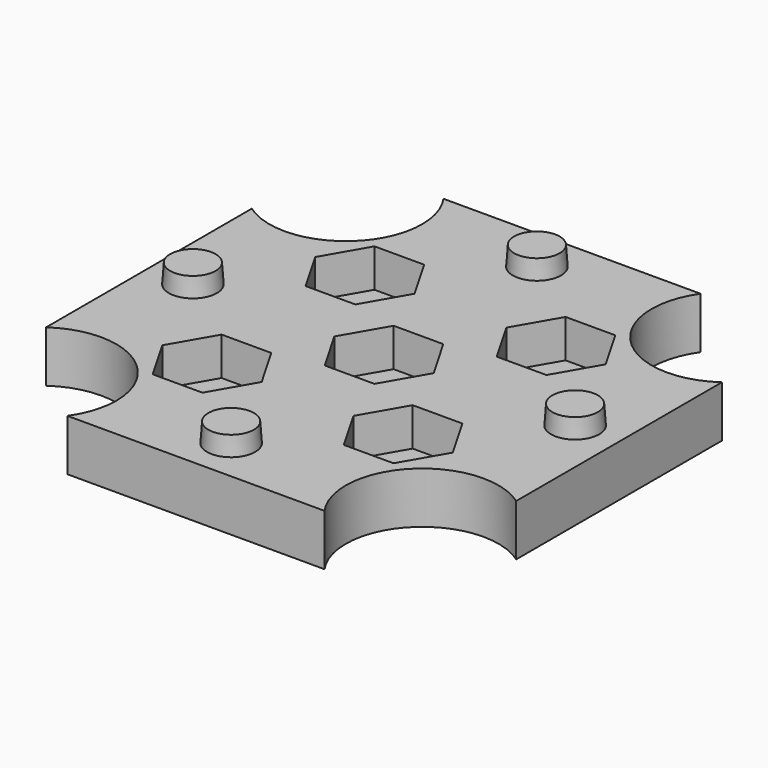
from build123d import *

# Parameters (mm, degrees)
F0_R       = 3.2004
F0_R_2     = 6.858
F1_DEPTH   = 6.8326
F2_DEPTH   = 9.3726
F3_R       = 3.2004
F4_DEPTH   = 5.08
F5_SIZE2   = 2.53999
F5_SIZE    = 0.17779
F5_2_SIZE2 = 2.53999
F5_2_SIZE  = 0.17779
F5_3_SIZE2 = 2.53999
F5_3_SIZE  = 0.17779
F5_4_SIZE2 = 2.53999
F5_4_SIZE  = 0.17779


# Not quite as in the source:
# - a fillet or chamfer is up to 0.001 mm smaller than in the source, because OpenCascade refuses the exact size


with BuildPart() as f1:
    # F0 (on Top) → F1 (new body)
    with BuildSketch(Plane.XY):
        with BuildLine():
            ThreePointArc((-31.242, -17.0875613686), (-20.7164714157, -16.3838944106), (-15.24, -25.4))
            ThreePointArc((-15.24, -25.4), (-15.712895776, -28.4635945803), (-17.0875613686, -31.242))
            Line((-17.0875613686, -31.242), (17.0875613686, -31.242))
            ThreePointArc((17.0875613686, -31.242), (18.2157951031, -18.2157951031), (31.242, -17.0875613686))
            Line((31.242, -17.0875613686), (31.242, 17.0875613686))
            ThreePointArc((31.242, 17.0875613686), (18.2157951031, 18.2157951031), (17.0875613686, 31.242))
            Line((17.0875613686, 31.242), (-17.0875613686, 31.242))
            ThreePointArc((-17.0875613686, 31.242), (-18.2157951031, 18.2157951031), (-31.242, 17.0875613686))
            Line((-31.242, 17.0875613686), (-31.242, -17.0875613686))
        make_face()
        with Locations((0, -25.4)):
            Circle(F0_R, mode=Mode.SUBTRACT)
        with Locations((-25.4, 0)):
            Circle(F0_R, mode=Mode.SUBTRACT)
        with Locations((-12.7, -12.7)):
            Circle(F0_R, mode=Mode.SUBTRACT)
        Circle(F0_R_2, mode=Mode.SUBTRACT)
        with Locations((12.7, -12.7)):
            Circle(F0_R, mode=Mode.SUBTRACT)
        with Locations((25.4, 0)):
            Circle(F0_R, mode=Mode.SUBTRACT)
        with Locations((-12.7, 12.7)):
            Circle(F0_R, mode=Mode.SUBTRACT)
        with Locations((0, 25.4)):
            Circle(F0_R, mode=Mode.SUBTRACT)
        with Locations((12.7, 12.7)):
            Circle(F0_R, mode=Mode.SUBTRACT)
        Circle(F0_R_2)
        Circle(F0_R, mode=Mode.SUBTRACT)
    extrude(amount=F1_DEPTH)

    # F0 (on Top) → F2 (join)
    with BuildSketch(Plane.XY):
        with Locations((-25.4, 0)):
            Circle(F0_R)
        with Locations((0, -25.4)):
            Circle(F0_R)
        with Locations((25.4, 0)):
            Circle(F0_R)
        with Locations((0, 25.4)):
            Circle(F0_R)
    extrude(amount=F2_DEPTH)

    # F3 (on face) → F4 (cut)
    with BuildSketch(Plane.XY.offset(6.8326)):
        Polygon((-9.398, 6.9807682334), (-6.096, 12.7), (-9.398, 18.4192317666), (-16.002, 18.4192317666), (-19.304, 12.7), (-16.002, 6.9807682334), align=None)
        with Locations((-12.7, 12.7)):
            Circle(F3_R, mode=Mode.SUBTRACT)
        Polygon((9.398, 18.4192317666), (6.096, 12.7), (9.398, 6.9807682334), (16.002, 6.9807682334), (19.304, 12.7), (16.002, 18.4192317666), align=None)
        with Locations((12.7, 12.7)):
            Circle(F3_R, mode=Mode.SUBTRACT)
        Polygon((-9.398, -18.4192317666), (-6.096, -12.7), (-9.398, -6.9807682334), (-16.002, -6.9807682334), (-19.304, -12.7), (-16.002, -18.4192317666), align=None)
        with Locations((-12.7, -12.7)):
            Circle(F3_R, mode=Mode.SUBTRACT)
        Polygon((9.398, -6.9807682334), (6.096, -12.7), (9.398, -18.4192317666), (16.002, -18.4192317666), (19.304, -12.7), (16.002, -6.9807682334), align=None)
        with Locations((12.7, -12.7)):
            Circle(F3_R, mode=Mode.SUBTRACT)
        Polygon((3.302, -5.7192317666), (6.604, 0), (3.302, 5.7192317666), (-3.302, 5.7192317666), (-6.604, 0), (-3.302, -5.7192317666), align=None)
        Circle(F3_R, mode=Mode.SUBTRACT)
    extrude(amount=-F4_DEPTH, mode=Mode.SUBTRACT)

    # F5 (size 0.1778 and 2.54 in the source; OpenCascade refuses exactly that, so slightly less here)
    f5_edges = [f1.edges().sort_by_distance(p)[0] for p in [
        (-28.6004, 0, 9.3726),
    ]]
    f5_side = f1.faces().sort_by_distance((-25.4, 0, 9.3726))[0]
    chamfer(f5_edges, length=F5_SIZE, length2=F5_SIZE2, reference=f5_side)

    # F5#2 (size 0.1778 and 2.54 in the source; OpenCascade refuses exactly that, so slightly less here)
    f5_2_edges = [f1.edges().sort_by_distance(p)[0] for p in [
        (-3.2004, 25.4, 9.3726),
    ]]
    f5_2_side = f1.faces().sort_by_distance((0, 25.4, 9.3726))[0]
    chamfer(f5_2_edges, length=F5_2_SIZE, length2=F5_2_SIZE2, reference=f5_2_side)

    # F5#3 (size 0.1778 and 2.54 in the source; OpenCascade refuses exactly that, so slightly less here)
    f5_3_edges = [f1.edges().sort_by_distance(p)[0] for p in [
        (22.1996, 0, 9.3726),
    ]]
    f5_3_side = f1.faces().sort_by_distance((25.4, 0, 9.3726))[0]
    chamfer(f5_3_edges, length=F5_3_SIZE, length2=F5_3_SIZE2, reference=f5_3_side)

    # F5#4 (size 0.1778 and 2.54 in the source; OpenCascade refuses exactly that, so slightly less here)
    f5_4_edges = [f1.edges().sort_by_distance(p)[0] for p in [
        (-3.2004, -25.4, 9.3726),
    ]]
    f5_4_side = f1.faces().sort_by_distance((0, -25.4, 9.3726))[0]
    chamfer(f5_4_edges, length=F5_4_SIZE, length2=F5_4_SIZE2, reference=f5_4_side)


solid = f1.part
